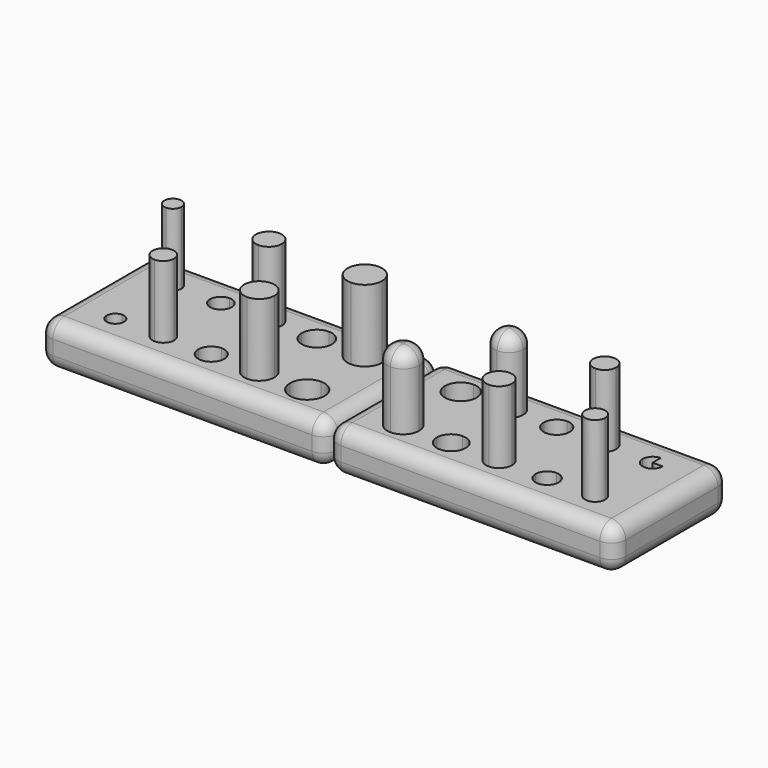
from build123d import *

# Parameters (mm, degrees)
F1_DEPTH = 3
F2_DEPTH = 5
F3_R     = 1
F4_DEPTH = 5
F5_DEPTH = 3
F6_R     = 1
F7_R     = 1


# Not quite as in the source:
# - a feature names something its author has since deleted; it is built from what else it names


with BuildPart() as f1:
    # F0 (on Top) → F1 (new body)
    with BuildSketch(Plane.XY):
        with BuildLine():
            Line((10, 0), (10, 2.5))
            Line((10, 2.5), (6.6666666667, 2.5))
            Line((6.6666666667, 2.5), (6.6666666667, 1.2))
            ThreePointArc((6.6666666667, 1.2), (7.5151948041, 0.8485281374), (7.8666666667, 0))
            Line((7.8666666667, 0), (10, 0))
        make_face()
        with BuildLine():
            Line((-6.6666666667, 0.6), (-6.6666666667, 2.5))
            Line((-6.6666666667, 2.5), (-10, 2.5))
            Line((-10, 2.5), (-10, 0))
            Line((-10, 0), (-7.2666666667, 0))
            ThreePointArc((-7.2666666667, 0), (-7.0909307354, 0.4242640687), (-6.6666666667, 0.6))
        make_face()
        with BuildLine():
            Line((10, -7.5), (10, -5))
            Line((10, -5), (7.8666666667, -5))
            ThreePointArc((7.8666666667, -5), (7.5151948041, -5.8485281374), (6.6666666667, -6.2))
            Line((6.6666666667, -6.2), (6.6666666667, -7.5))
            Line((6.6666666667, -7.5), (10, -7.5))
        make_face()
        with BuildLine():
            Line((-7.2666666667, -5), (-10, -5))
            Line((-10, -5), (-10, -7.5))
            Line((-10, -7.5), (-6.6666666667, -7.5))
            Line((-6.6666666667, -7.5), (-6.6666666667, -5.6))
            ThreePointArc((-6.6666666667, -5.6), (-7.0909307354, -5.4242640687), (-7.2666666667, -5))
        make_face()
        with BuildLine():
            Line((10, -2.5), (10, 0))
            Line((10, 0), (7.8666666667, 0))
            ThreePointArc((7.8666666667, 0), (7.5151948041, -0.8485281374), (6.6666666667, -1.2))
            Line((6.6666666667, -1.2), (6.6666666667, -2.5))
            Line((6.6666666667, -2.5), (10, -2.5))
        make_face()
        with BuildLine():
            Line((10, -5), (10, -2.5))
            Line((10, -2.5), (6.6666666667, -2.5))
            Line((6.6666666667, -2.5), (6.6666666667, -3.8))
            ThreePointArc((6.6666666667, -3.8), (7.5151948041, -4.1514718626), (7.8666666667, -5))
            Line((7.8666666667, -5), (10, -5))
        make_face()
        with BuildLine():
            Line((-7.2666666667, 0), (-10, 0))
            Line((-10, 0), (-10, -2.5))
            Line((-10, -2.5), (-6.6666666667, -2.5))
            Line((-6.6666666667, -2.5), (-6.6666666667, -0.6))
            ThreePointArc((-6.6666666667, -0.6), (-7.0909307354, -0.4242640687), (-7.2666666667, 0))
        make_face()
        with BuildLine():
            Line((-6.6666666667, -4.4), (-6.6666666667, -2.5))
            Line((-6.6666666667, -2.5), (-10, -2.5))
            Line((-10, -2.5), (-10, -5))
            Line((-10, -5), (-7.2666666667, -5))
            ThreePointArc((-7.2666666667, -5), (-7.0909307354, -4.5757359313), (-6.6666666667, -4.4))
        make_face()
        with BuildLine():
            Line((6.6666666667, 1.2), (6.6666666667, 2.5))
            Line((6.6666666667, 2.5), (3.3333333333, 2.5))
            Line((3.3333333333, 2.5), (3.3333333333, 1.05))
            ThreePointArc((3.3333333333, 1.05), (4.0757954536, 0.7424621202), (4.3833333333, 0))
            Line((4.3833333333, 0), (5.4666666667, 0))
            ThreePointArc((5.4666666667, 0), (5.8181385292, 0.8485281374), (6.6666666667, 1.2))
        make_face()
        with BuildLine():
            Line((3.3333333333, 1.05), (3.3333333333, 2.5))
            Line((3.3333333333, 2.5), (0, 2.5))
            Line((0, 2.5), (0, 0.9))
            ThreePointArc((0, 0.9), (0.6363961031, 0.6363961031), (0.9, 0))
            Line((0.9, 0), (2.2833333333, 0))
            ThreePointArc((2.2833333333, 0), (2.5908712131, 0.7424621202), (3.3333333333, 1.05))
        make_face()
        with BuildLine():
            Line((0, 0.9), (0, 2.5))
            Line((0, 2.5), (-3.3333333333, 2.5))
            Line((-3.3333333333, 2.5), (-3.3333333333, 0.75))
            ThreePointArc((-3.3333333333, 0.75), (-2.8030032474, 0.5303300859), (-2.5833333333, 0))
            Line((-2.5833333333, 0), (-0.9, 0))
            ThreePointArc((-0.9, 0), (-0.6363961031, 0.6363961031), (0, 0.9))
        make_face()
        with BuildLine():
            Line((-3.3333333333, 0.75), (-3.3333333333, 2.5))
            Line((-3.3333333333, 2.5), (-6.6666666667, 2.5))
            Line((-6.6666666667, 2.5), (-6.6666666667, 0.6))
            ThreePointArc((-6.6666666667, 0.6), (-6.242402598, 0.4242640687), (-6.0666666667, 0))
            Line((-6.0666666667, 0), (-4.0833333333, 0))
            ThreePointArc((-4.0833333333, 0), (-3.8636634192, 0.5303300859), (-3.3333333333, 0.75))
        make_face()
        with BuildLine():
            ThreePointArc((3.3333333333, -6.05), (2.5908712131, -5.7424621202), (2.2833333333, -5))
            Line((2.2833333333, -5), (0.9, -5))
            ThreePointArc((0.9, -5), (0.6363961031, -5.6363961031), (0, -5.9))
            Line((0, -5.9), (0, -7.5))
            Line((0, -7.5), (3.3333333333, -7.5))
            Line((3.3333333333, -7.5), (3.3333333333, -6.05))
        make_face()
        with BuildLine():
            ThreePointArc((-3.3333333333, -5.75), (-3.8636634192, -5.5303300859), (-4.0833333333, -5))
            Line((-4.0833333333, -5), (-6.0666666667, -5))
            ThreePointArc((-6.0666666667, -5), (-6.242402598, -5.4242640687), (-6.6666666667, -5.6))
            Line((-6.6666666667, -5.6), (-6.6666666667, -7.5))
            Line((-6.6666666667, -7.5), (-3.3333333333, -7.5))
            Line((-3.3333333333, -7.5), (-3.3333333333, -5.75))
        make_face()
        with BuildLine():
            ThreePointArc((6.6666666667, -1.2), (5.8181385292, -0.8485281374), (5.4666666667, 0))
            Line((5.4666666667, 0), (4.3833333333, 0))
            ThreePointArc((4.3833333333, 0), (4.0757954536, -0.7424621202), (3.3333333333, -1.05))
            Line((3.3333333333, -1.05), (3.3333333333, -2.5))
            Line((3.3333333333, -2.5), (6.6666666667, -2.5))
            Line((6.6666666667, -2.5), (6.6666666667, -1.2))
        make_face()
        with BuildLine():
            ThreePointArc((3.3333333333, -1.05), (2.5908712131, -0.7424621202), (2.2833333333, 0))
            Line((2.2833333333, 0), (0.9, 0))
            ThreePointArc((0.9, 0), (0.6363961031, -0.6363961031), (0, -0.9))
            Line((0, -0.9), (0, -2.5))
            Line((0, -2.5), (3.3333333333, -2.5))
            Line((3.3333333333, -2.5), (3.3333333333, -1.05))
        make_face()
        with BuildLine():
            ThreePointArc((0, -0.9), (-0.6363961031, -0.6363961031), (-0.9, 0))
            Line((-0.9, 0), (-2.5833333333, 0))
            ThreePointArc((-2.5833333333, 0), (-2.8030032474, -0.5303300859), (-3.3333333333, -0.75))
            Line((-3.3333333333, -0.75), (-3.3333333333, -2.5))
            Line((-3.3333333333, -2.5), (0, -2.5))
            Line((0, -2.5), (0, -0.9))
        make_face()
        with BuildLine():
            ThreePointArc((-3.3333333333, -0.75), (-3.8636634192, -0.5303300859), (-4.0833333333, 0))
            Line((-4.0833333333, 0), (-6.0666666667, 0))
            ThreePointArc((-6.0666666667, 0), (-6.242402598, -0.4242640687), (-6.6666666667, -0.6))
            Line((-6.6666666667, -0.6), (-6.6666666667, -2.5))
            Line((-6.6666666667, -2.5), (-3.3333333333, -2.5))
            Line((-3.3333333333, -2.5), (-3.3333333333, -0.75))
        make_face()
        with BuildLine():
            Line((0, -4.1), (0, -2.5))
            Line((0, -2.5), (-3.3333333333, -2.5))
            Line((-3.3333333333, -2.5), (-3.3333333333, -4.25))
            ThreePointArc((-3.3333333333, -4.25), (-2.8030032474, -4.4696699141), (-2.5833333333, -5))
            Line((-2.5833333333, -5), (-0.9, -5))
            ThreePointArc((-0.9, -5), (-0.6363961031, -4.3636038969), (0, -4.1))
        make_face()
        with BuildLine():
            Line((3.3333333333, -3.95), (3.3333333333, -2.5))
            Line((3.3333333333, -2.5), (0, -2.5))
            Line((0, -2.5), (0, -4.1))
            ThreePointArc((0, -4.1), (0.6363961031, -4.3636038969), (0.9, -5))
            Line((0.9, -5), (2.2833333333, -5))
            ThreePointArc((2.2833333333, -5), (2.5908712131, -4.2575378798), (3.3333333333, -3.95))
        make_face()
        with BuildLine():
            Line((6.6666666667, -3.8), (6.6666666667, -2.5))
            Line((6.6666666667, -2.5), (3.3333333333, -2.5))
            Line((3.3333333333, -2.5), (3.3333333333, -3.95))
            ThreePointArc((3.3333333333, -3.95), (4.0757954536, -4.2575378798), (4.3833333333, -5))
            Line((4.3833333333, -5), (5.4666666667, -5))
            ThreePointArc((5.4666666667, -5), (5.8181385292, -4.1514718626), (6.6666666667, -3.8))
        make_face()
        with BuildLine():
            ThreePointArc((6.6666666667, -6.2), (5.8181385292, -5.8485281374), (5.4666666667, -5))
            Line((5.4666666667, -5), (4.3833333333, -5))
            ThreePointArc((4.3833333333, -5), (4.0757954536, -5.7424621202), (3.3333333333, -6.05))
            Line((3.3333333333, -6.05), (3.3333333333, -7.5))
            Line((3.3333333333, -7.5), (6.6666666667, -7.5))
            Line((6.6666666667, -7.5), (6.6666666667, -6.2))
        make_face()
        with BuildLine():
            ThreePointArc((0, -5.9), (-0.6363961031, -5.6363961031), (-0.9, -5))
            Line((-0.9, -5), (-2.5833333333, -5))
            ThreePointArc((-2.5833333333, -5), (-2.8030032474, -5.5303300859), (-3.3333333333, -5.75))
            Line((-3.3333333333, -5.75), (-3.3333333333, -7.5))
            Line((-3.3333333333, -7.5), (0, -7.5))
            Line((0, -7.5), (0, -5.9))
        make_face()
        with BuildLine():
            Line((-6.6666666667, -0.6), (-6.6666666667, 0))
            Line((-6.6666666667, 0), (-7.2666666667, 0))
            ThreePointArc((-7.2666666667, 0), (-7.0909307354, -0.4242640687), (-6.6666666667, -0.6))
        make_face()
        with BuildLine():
            Line((-6.0666666667, 0), (-6.6666666667, 0))
            Line((-6.6666666667, 0), (-6.6666666667, -0.6))
            ThreePointArc((-6.6666666667, -0.6), (-6.242402598, -0.4242640687), (-6.0666666667, 0))
        make_face()
        with BuildLine():
            ThreePointArc((-6.0666666667, 0), (-6.242402598, 0.4242640687), (-6.6666666667, 0.6))
            Line((-6.6666666667, 0.6), (-6.6666666667, 0))
            Line((-6.6666666667, 0), (-6.0666666667, 0))
        make_face()
        with BuildLine():
            Line((-6.6666666667, 0), (-6.6666666667, 0.6))
            ThreePointArc((-6.6666666667, 0.6), (-7.0909307354, 0.4242640687), (-7.2666666667, 0))
            Line((-7.2666666667, 0), (-6.6666666667, 0))
        make_face()
        with BuildLine():
            Line((0, 0), (0, 0.9))
            ThreePointArc((0, 0.9), (-0.6363961031, 0.6363961031), (-0.9, 0))
            Line((-0.9, 0), (0, 0))
        make_face()
        with BuildLine():
            ThreePointArc((0, -0.9), (0.6363961031, -0.6363961031), (0.9, 0))
            Line((0.9, 0), (0, 0))
            Line((0, 0), (0, -0.9))
        make_face()
        with BuildLine():
            ThreePointArc((0.9, 0), (0.6363961031, 0.6363961031), (0, 0.9))
            Line((0, 0.9), (0, 0))
            Line((0, 0), (0.9, 0))
        make_face()
        with BuildLine():
            ThreePointArc((7.8666666667, 0), (7.5151948041, 0.8485281374), (6.6666666667, 1.2))
            Line((6.6666666667, 1.2), (6.6666666667, 0))
            Line((6.6666666667, 0), (7.8666666667, 0))
        make_face()
        with BuildLine():
            ThreePointArc((6.6666666667, -1.2), (7.5151948041, -0.8485281374), (7.8666666667, 0))
            Line((7.8666666667, 0), (6.6666666667, 0))
            Line((6.6666666667, 0), (6.6666666667, -1.2))
        make_face()
        with BuildLine():
            Line((6.6666666667, -1.2), (6.6666666667, 0))
            Line((6.6666666667, 0), (5.4666666667, 0))
            ThreePointArc((5.4666666667, 0), (5.8181385292, -0.8485281374), (6.6666666667, -1.2))
        make_face()
        with BuildLine():
            Line((6.6666666667, 0), (6.6666666667, 1.2))
            ThreePointArc((6.6666666667, 1.2), (5.8181385292, 0.8485281374), (5.4666666667, 0))
            Line((5.4666666667, 0), (6.6666666667, 0))
        make_face()
        with BuildLine():
            Line((0, 0), (-0.9, 0))
            ThreePointArc((-0.9, 0), (-0.6363961031, -0.6363961031), (0, -0.9))
            Line((0, -0.9), (0, 0))
        make_face()
        with BuildLine():
            Line((3.3333333333, -6.05), (3.3333333333, -5))
            Line((3.3333333333, -5), (2.2833333333, -5))
            ThreePointArc((2.2833333333, -5), (2.5908712131, -5.7424621202), (3.3333333333, -6.05))
        make_face()
        with BuildLine():
            Line((3.3333333333, -5), (3.3333333333, -3.95))
            ThreePointArc((3.3333333333, -3.95), (2.5908712131, -4.2575378798), (2.2833333333, -5))
            Line((2.2833333333, -5), (3.3333333333, -5))
        make_face()
        with BuildLine():
            ThreePointArc((4.3833333333, -5), (4.0757954536, -4.2575378798), (3.3333333333, -3.95))
            Line((3.3333333333, -3.95), (3.3333333333, -5))
            Line((3.3333333333, -5), (4.3833333333, -5))
        make_face()
        with BuildLine():
            Line((4.3833333333, -5), (3.3333333333, -5))
            Line((3.3333333333, -5), (3.3333333333, -6.05))
            ThreePointArc((3.3333333333, -6.05), (4.0757954536, -5.7424621202), (4.3833333333, -5))
        make_face()
        with BuildLine():
            Line((-2.5833333333, -5), (-3.3333333333, -5))
            Line((-3.3333333333, -5), (-3.3333333333, -5.75))
            ThreePointArc((-3.3333333333, -5.75), (-2.8030032474, -5.5303300859), (-2.5833333333, -5))
        make_face()
        with BuildLine():
            Line((-3.3333333333, -5.75), (-3.3333333333, -5))
            Line((-3.3333333333, -5), (-4.0833333333, -5))
            ThreePointArc((-4.0833333333, -5), (-3.8636634192, -5.5303300859), (-3.3333333333, -5.75))
        make_face()
        with BuildLine():
            ThreePointArc((-2.5833333333, -5), (-2.8030032474, -4.4696699141), (-3.3333333333, -4.25))
            Line((-3.3333333333, -4.25), (-3.3333333333, -5))
            Line((-3.3333333333, -5), (-2.5833333333, -5))
        make_face()
        with BuildLine():
            Line((-3.3333333333, -4.25), (-3.3333333333, -2.5))
            Line((-3.3333333333, -2.5), (-6.6666666667, -2.5))
            Line((-6.6666666667, -2.5), (-6.6666666667, -4.4))
            ThreePointArc((-6.6666666667, -4.4), (-6.242402598, -4.5757359313), (-6.0666666667, -5))
            Line((-6.0666666667, -5), (-4.0833333333, -5))
            ThreePointArc((-4.0833333333, -5), (-3.8636634192, -4.4696699141), (-3.3333333333, -4.25))
        make_face()
        with BuildLine():
            Line((-3.3333333333, -5), (-3.3333333333, -4.25))
            ThreePointArc((-3.3333333333, -4.25), (-3.8636634192, -4.4696699141), (-4.0833333333, -5))
            Line((-4.0833333333, -5), (-3.3333333333, -5))
        make_face()
    extrude(amount=-F1_DEPTH)

    # F0 (on Top) → F2 (join)
    with BuildSketch(Plane.XY):
        with BuildLine():
            Line((0, 0), (-0.9, 0))
            ThreePointArc((-0.9, 0), (-0.6363961031, -0.6363961031), (0, -0.9))
            Line((0, -0.9), (0, 0))
        make_face()
        with BuildLine():
            Line((0, 0), (0, 0.9))
            ThreePointArc((0, 0.9), (-0.6363961031, 0.6363961031), (-0.9, 0))
            Line((-0.9, 0), (0, 0))
        make_face()
        with BuildLine():
            ThreePointArc((0, -0.9), (0.6363961031, -0.6363961031), (0.9, 0))
            Line((0.9, 0), (0, 0))
            Line((0, 0), (0, -0.9))
        make_face()
        with BuildLine():
            ThreePointArc((0.9, 0), (0.6363961031, 0.6363961031), (0, 0.9))
            Line((0, 0.9), (0, 0))
            Line((0, 0), (0.9, 0))
        make_face()
        with BuildLine():
            ThreePointArc((-2.5833333333, -5), (-2.8030032474, -4.4696699141), (-3.3333333333, -4.25))
            Line((-3.3333333333, -4.25), (-3.3333333333, -5))
            Line((-3.3333333333, -5), (-2.5833333333, -5))
        make_face()
        with BuildLine():
            Line((-2.5833333333, -5), (-3.3333333333, -5))
            Line((-3.3333333333, -5), (-3.3333333333, -5.75))
            ThreePointArc((-3.3333333333, -5.75), (-2.8030032474, -5.5303300859), (-2.5833333333, -5))
        make_face()
        with BuildLine():
            Line((-3.3333333333, -5.75), (-3.3333333333, -5))
            Line((-3.3333333333, -5), (-4.0833333333, -5))
            ThreePointArc((-4.0833333333, -5), (-3.8636634192, -5.5303300859), (-3.3333333333, -5.75))
        make_face()
        with BuildLine():
            Line((-3.3333333333, -5), (-3.3333333333, -4.25))
            ThreePointArc((-3.3333333333, -4.25), (-3.8636634192, -4.4696699141), (-4.0833333333, -5))
            Line((-4.0833333333, -5), (-3.3333333333, -5))
        make_face()
        with BuildLine():
            ThreePointArc((-6.0666666667, 0), (-6.242402598, 0.4242640687), (-6.6666666667, 0.6))
            Line((-6.6666666667, 0.6), (-6.6666666667, 0))
            Line((-6.6666666667, 0), (-6.0666666667, 0))
        make_face()
        with BuildLine():
            Line((-6.6666666667, 0), (-6.6666666667, 0.6))
            ThreePointArc((-6.6666666667, 0.6), (-7.0909307354, 0.4242640687), (-7.2666666667, 0))
            Line((-7.2666666667, 0), (-6.6666666667, 0))
        make_face()
        with BuildLine():
            Line((-6.6666666667, -0.6), (-6.6666666667, 0))
            Line((-6.6666666667, 0), (-7.2666666667, 0))
            ThreePointArc((-7.2666666667, 0), (-7.0909307354, -0.4242640687), (-6.6666666667, -0.6))
        make_face()
        with BuildLine():
            Line((-6.0666666667, 0), (-6.6666666667, 0))
            Line((-6.6666666667, 0), (-6.6666666667, -0.6))
            ThreePointArc((-6.6666666667, -0.6), (-6.242402598, -0.4242640687), (-6.0666666667, 0))
        make_face()
        with BuildLine():
            Line((3.3333333333, -5), (3.3333333333, -3.95))
            ThreePointArc((3.3333333333, -3.95), (2.5908712131, -4.2575378798), (2.2833333333, -5))
            Line((2.2833333333, -5), (3.3333333333, -5))
        make_face()
        with BuildLine():
            Line((3.3333333333, -6.05), (3.3333333333, -5))
            Line((3.3333333333, -5), (2.2833333333, -5))
            ThreePointArc((2.2833333333, -5), (2.5908712131, -5.7424621202), (3.3333333333, -6.05))
        make_face()
        with BuildLine():
            Line((4.3833333333, -5), (3.3333333333, -5))
            Line((3.3333333333, -5), (3.3333333333, -6.05))
            ThreePointArc((3.3333333333, -6.05), (4.0757954536, -5.7424621202), (4.3833333333, -5))
        make_face()
        with BuildLine():
            ThreePointArc((4.3833333333, -5), (4.0757954536, -4.2575378798), (3.3333333333, -3.95))
            Line((3.3333333333, -3.95), (3.3333333333, -5))
            Line((3.3333333333, -5), (4.3833333333, -5))
        make_face()
        with BuildLine():
            Line((6.6666666667, -1.2), (6.6666666667, 0))
            Line((6.6666666667, 0), (5.4666666667, 0))
            ThreePointArc((5.4666666667, 0), (5.8181385292, -0.8485281374), (6.6666666667, -1.2))
        make_face()
        with BuildLine():
            Line((6.6666666667, 0), (6.6666666667, 1.2))
            ThreePointArc((6.6666666667, 1.2), (5.8181385292, 0.8485281374), (5.4666666667, 0))
            Line((5.4666666667, 0), (6.6666666667, 0))
        make_face()
        with BuildLine():
            ThreePointArc((7.8666666667, 0), (7.5151948041, 0.8485281374), (6.6666666667, 1.2))
            Line((6.6666666667, 1.2), (6.6666666667, 0))
            Line((6.6666666667, 0), (7.8666666667, 0))
        make_face()
        with BuildLine():
            ThreePointArc((6.6666666667, -1.2), (7.5151948041, -0.8485281374), (7.8666666667, 0))
            Line((7.8666666667, 0), (6.6666666667, 0))
            Line((6.6666666667, 0), (6.6666666667, -1.2))
        make_face()
    extrude(amount=F2_DEPTH)

    # F3
    f3_edges = [f1.edges().sort_by_distance(p)[0] for p in [
        (-10, 2.5, -1.5),
        (-10, -7.5, -1.5),
        (-10, -2.5, 0),
        (-10, -2.5, -3),
        (10, -7.5, -1.5),
        (0, -7.5, 0),
        (0, -7.5, -3),
        (10, 2.5, -1.5),
        (0, 2.5, 0),
        (0, 2.5, -3),
        (10, -2.5, 0),
        (10, -2.5, -3),
    ]]
    fillet(f3_edges, radius=F3_R)


with BuildPart() as f4:
    # F0 (on Top) → F4 (new body)
    with BuildSketch(Plane.XY):
        with BuildLine():
            ThreePointArc((24.1333333333, 0), (23.8990187583, 0.5656854249), (23.3333333333, 0.8))
            ThreePointArc((23.3333333333, 0.8), (22.7676479084, 0.5656854249), (22.5333333333, 0))
            ThreePointArc((22.5333333333, 0), (22.7676479084, -0.5656854249), (23.3333333333, -0.8))
            ThreePointArc((23.3333333333, -0.8), (23.8990187583, -0.5656854249), (24.1333333333, 0))
        make_face()
    extrude(amount=F4_DEPTH)



with BuildPart() as f4b:
    # F0 (on Top) → F4, piece 2 (new body)
    with BuildSketch(Plane.XY):
        with BuildLine():
            ThreePointArc((20.9, -5), (20.6363961031, -4.3636038969), (20, -4.1))
            ThreePointArc((20, -4.1), (19.3636038969, -4.3636038969), (19.1, -5))
            ThreePointArc((19.1, -5), (19.3636038969, -5.6363961031), (20, -5.9))
            ThreePointArc((20, -5.9), (20.6363961031, -5.6363961031), (20.9, -5))
        make_face()
    extrude(amount=F4_DEPTH)


with BuildPart() as f4c:
    # F0 (on Top) → F4, piece 3 (new body)
    with BuildSketch(Plane.XY):
        with BuildLine():
            ThreePointArc((17.6666666667, 0), (17.3737734479, 0.7071067812), (16.6666666667, 1))
            ThreePointArc((16.6666666667, 1), (15.6666666667, 0), (16.6666666667, -1))
            ThreePointArc((16.6666666667, -1), (17.3737734479, -0.7071067812), (17.6666666667, 0))
        make_face()
    extrude(amount=F4_DEPTH)


with BuildPart() as f4d:
    # F0 (on Top) → F4, piece 4 (new body)
    with BuildSketch(Plane.XY):
        with BuildLine():
            ThreePointArc((13.3333333333, -3.9), (12.555515874, -4.2221825407), (12.2333333333, -5))
            ThreePointArc((12.2333333333, -5), (12.555515874, -5.7778174593), (13.3333333333, -6.1))
            ThreePointArc((13.3333333333, -6.1), (14.1111507926, -5.7778174593), (14.4333333333, -5))
            ThreePointArc((14.4333333333, -5), (14.1111507926, -4.2221825407), (13.3333333333, -3.9))
        make_face()
    extrude(amount=F4_DEPTH)


with BuildPart() as f4e:
    # F0 (on Top) → F4, piece 5 (new body)
    with BuildSketch(Plane.XY):
        with BuildLine():
            ThreePointArc((27.3666666667, -5), (27.1616414135, -4.5050252532), (26.6666666667, -4.3))
            ThreePointArc((26.6666666667, -4.3), (26.1716919198, -4.5050252532), (25.9666666667, -5))
            ThreePointArc((25.9666666667, -5), (26.6666666667, -5.7), (27.3666666667, -5))
        make_face()
    extrude(amount=F4_DEPTH)


with BuildPart() as f4_1:
    add(f4.part)

    add(f4b.part)  # F5 merges F4b

    add(f4c.part)  # F5 merges F4c

    add(f4d.part)  # F5 merges F4d

    add(f4e.part)  # F5 merges F4e
    # F0 (on Top) → F5 (join)
    with BuildSketch(Plane.XY):
        with BuildLine():
            Line((23.3333333333, 2.5), (20, 2.5))
            Line((20, 2.5), (20, 0.9))
            ThreePointArc((20, 0.9), (20.6363961031, 0.6363961031), (20.9, 0))
            Line((20.9, 0), (22.5333333333, 0))
            ThreePointArc((22.5333333333, 0), (22.7676479084, 0.5656854249), (23.3333333333, 0.8))
            Line((23.3333333333, 0.8), (23.3333333333, 2.5))
        make_face()
        with BuildLine():
            Line((12.2333333333, -5), (10, -5))
            Line((10, -5), (10, -7.5))
            Line((10, -7.5), (13.3333333333, -7.5))
            Line((13.3333333333, -7.5), (13.3333333333, -6.1))
            ThreePointArc((13.3333333333, -6.1), (12.555515874, -5.7778174593), (12.2333333333, -5))
        make_face()
        with BuildLine():
            Line((16.6666666667, -2.5), (13.3333333333, -2.5))
            Line((13.3333333333, -2.5), (13.3333333333, -3.9))
            ThreePointArc((13.3333333333, -3.9), (14.1111507926, -4.2221825407), (14.4333333333, -5))
            Line((14.4333333333, -5), (15.6666666667, -5))
            ThreePointArc((15.6666666667, -5), (15.9595598855, -4.2928932188), (16.6666666667, -4))
            Line((16.6666666667, -4), (16.6666666667, -2.5))
        make_face()
        with BuildLine():
            Line((20, -5.9), (20, -7.5))
            Line((20, -7.5), (30, -7.5))
            Line((30, -7.5), (30, -5))
            Line((30, -5), (27.3666666667, -5))
            ThreePointArc((27.3666666667, -5), (26.6666666667, -5.7), (25.9666666667, -5))
            Line((25.9666666667, -5), (24.1333333333, -5))
            ThreePointArc((24.1333333333, -5), (23.3333333333, -5.8), (22.5333333333, -5))
            Line((22.5333333333, -5), (20.9, -5))
            ThreePointArc((20.9, -5), (20.6363961031, -5.6363961031), (20, -5.9))
        make_face()
        with BuildLine():
            Line((12.2333333333, 0), (10, 0))
            Line((10, 0), (10, -2.5))
            Line((10, -2.5), (13.3333333333, -2.5))
            Line((13.3333333333, -2.5), (13.3333333333, -1.1))
            ThreePointArc((13.3333333333, -1.1), (12.555515874, -0.7778174593), (12.2333333333, 0))
        make_face()
        with BuildLine():
            ThreePointArc((27.3666666667, 0), (27.1616414135, 0.4949747468), (26.6666666667, 0.7))
            Line((26.6666666667, 0.7), (26.6666666667, 0))
            Line((26.6666666667, 0), (27.3666666667, 0))
        make_face()
        with BuildLine():
            ThreePointArc((20.9, -5), (20.6363961031, -4.3636038969), (20, -4.1))
            ThreePointArc((20, -4.1), (19.3636038969, -4.3636038969), (19.1, -5))
            ThreePointArc((19.1, -5), (19.3636038969, -5.6363961031), (20, -5.9))
            ThreePointArc((20, -5.9), (20.6363961031, -5.6363961031), (20.9, -5))
        make_face()
        with BuildLine():
            Line((13.3333333333, -2.5), (10, -2.5))
            Line((10, -2.5), (10, -5))
            Line((10, -5), (12.2333333333, -5))
            ThreePointArc((12.2333333333, -5), (12.555515874, -4.2221825407), (13.3333333333, -3.9))
            Line((13.3333333333, -3.9), (13.3333333333, -2.5))
        make_face()
        with BuildLine():
            Line((30, -2.5), (26.6666666667, -2.5))
            Line((26.6666666667, -2.5), (26.6666666667, -4.3))
            ThreePointArc((26.6666666667, -4.3), (27.1616414135, -4.5050252532), (27.3666666667, -5))
            Line((27.3666666667, -5), (30, -5))
            Line((30, -5), (30, -2.5))
        make_face()
        with BuildLine():
            Line((23.3333333333, -0.8), (23.3333333333, -2.5))
            Line((23.3333333333, -2.5), (26.6666666667, -2.5))
            Line((26.6666666667, -2.5), (30, -2.5))
            Line((30, -2.5), (30, 0))
            Line((30, 0), (27.3666666667, 0))
            ThreePointArc((27.3666666667, 0), (26.6666666667, -0.7), (25.9666666667, 0))
            Line((25.9666666667, 0), (24.1333333333, 0))
            ThreePointArc((24.1333333333, 0), (23.8990187583, -0.5656854249), (23.3333333333, -0.8))
        make_face()
        with BuildLine():
            Line((16.6666666667, -6), (16.6666666667, -7.5))
            Line((16.6666666667, -7.5), (20, -7.5))
            Line((20, -7.5), (20, -5.9))
            ThreePointArc((20, -5.9), (19.3636038969, -5.6363961031), (19.1, -5))
            Line((19.1, -5), (17.6666666667, -5))
            ThreePointArc((17.6666666667, -5), (17.3737734479, -5.7071067812), (16.6666666667, -6))
        make_face()
        with BuildLine():
            ThreePointArc((24.1333333333, 0), (23.8990187583, 0.5656854249), (23.3333333333, 0.8))
            ThreePointArc((23.3333333333, 0.8), (22.7676479084, 0.5656854249), (22.5333333333, 0))
            ThreePointArc((22.5333333333, 0), (22.7676479084, -0.5656854249), (23.3333333333, -0.8))
            ThreePointArc((23.3333333333, -0.8), (23.8990187583, -0.5656854249), (24.1333333333, 0))
        make_face()
        with BuildLine():
            ThreePointArc((17.6666666667, 0), (17.3737734479, 0.7071067812), (16.6666666667, 1))
            ThreePointArc((16.6666666667, 1), (15.6666666667, 0), (16.6666666667, -1))
            ThreePointArc((16.6666666667, -1), (17.3737734479, -0.7071067812), (17.6666666667, 0))
        make_face()
        with BuildLine():
            Line((13.3333333333, -6.1), (13.3333333333, -7.5))
            Line((13.3333333333, -7.5), (16.6666666667, -7.5))
            Line((16.6666666667, -7.5), (16.6666666667, -6))
            ThreePointArc((16.6666666667, -6), (15.9595598855, -5.7071067812), (15.6666666667, -5))
            Line((15.6666666667, -5), (14.4333333333, -5))
            ThreePointArc((14.4333333333, -5), (14.1111507926, -5.7778174593), (13.3333333333, -6.1))
        make_face()
        with BuildLine():
            Line((26.6666666667, -2.5), (23.3333333333, -2.5))
            Line((23.3333333333, -2.5), (23.3333333333, -4.2))
            ThreePointArc((23.3333333333, -4.2), (23.8990187583, -4.4343145751), (24.1333333333, -5))
            Line((24.1333333333, -5), (25.9666666667, -5))
            ThreePointArc((25.9666666667, -5), (26.1716919198, -4.5050252532), (26.6666666667, -4.3))
            Line((26.6666666667, -4.3), (26.6666666667, -2.5))
        make_face()
        with BuildLine():
            Line((16.6666666667, -1), (16.6666666667, -2.5))
            Line((16.6666666667, -2.5), (20, -2.5))
            Line((20, -2.5), (20, -0.9))
            ThreePointArc((20, -0.9), (19.3636038969, -0.6363961031), (19.1, 0))
            Line((19.1, 0), (17.6666666667, 0))
            ThreePointArc((17.6666666667, 0), (17.3737734479, -0.7071067812), (16.6666666667, -1))
        make_face()
        with BuildLine():
            Line((23.3333333333, -2.5), (20, -2.5))
            Line((20, -2.5), (20, -4.1))
            ThreePointArc((20, -4.1), (20.6363961031, -4.3636038969), (20.9, -5))
            Line((20.9, -5), (22.5333333333, -5))
            ThreePointArc((22.5333333333, -5), (22.7676479084, -4.4343145751), (23.3333333333, -4.2))
            Line((23.3333333333, -4.2), (23.3333333333, -2.5))
        make_face()
        with BuildLine():
            Line((26.6666666667, 2.5), (23.3333333333, 2.5))
            Line((23.3333333333, 2.5), (23.3333333333, 0.8))
            ThreePointArc((23.3333333333, 0.8), (23.8990187583, 0.5656854249), (24.1333333333, 0))
            Line((24.1333333333, 0), (25.9666666667, 0))
            ThreePointArc((25.9666666667, 0), (26.1716919198, 0.4949747468), (26.6666666667, 0.7))
            Line((26.6666666667, 0.7), (26.6666666667, 2.5))
        make_face()
        with BuildLine():
            Line((30, 2.5), (26.6666666667, 2.5))
            Line((26.6666666667, 2.5), (26.6666666667, 0.7))
            ThreePointArc((26.6666666667, 0.7), (27.1616414135, 0.4949747468), (27.3666666667, 0))
            Line((27.3666666667, 0), (30, 0))
            Line((30, 0), (30, 2.5))
        make_face()
        with BuildLine():
            Line((16.6666666667, 2.5), (13.3333333333, 2.5))
            Line((13.3333333333, 2.5), (13.3333333333, 1.1))
            ThreePointArc((13.3333333333, 1.1), (14.1111507926, 0.7778174593), (14.4333333333, 0))
            ThreePointArc((14.4333333333, 0), (14.1111507926, -0.7778174593), (13.3333333333, -1.1))
            Line((13.3333333333, -1.1), (13.3333333333, -2.5))
            Line((13.3333333333, -2.5), (16.6666666667, -2.5))
            Line((16.6666666667, -2.5), (16.6666666667, -1))
            ThreePointArc((16.6666666667, -1), (15.6666666667, 0), (16.6666666667, 1))
            Line((16.6666666667, 1), (16.6666666667, 2.5))
        make_face()
        with BuildLine():
            Line((20, -2.5), (16.6666666667, -2.5))
            Line((16.6666666667, -2.5), (16.6666666667, -4))
            ThreePointArc((16.6666666667, -4), (17.3737734479, -4.2928932188), (17.6666666667, -5))
            Line((17.6666666667, -5), (19.1, -5))
            ThreePointArc((19.1, -5), (19.3636038969, -4.3636038969), (20, -4.1))
            Line((20, -4.1), (20, -2.5))
        make_face()
        with BuildLine():
            ThreePointArc((27.3666666667, -5), (27.1616414135, -4.5050252532), (26.6666666667, -4.3))
            ThreePointArc((26.6666666667, -4.3), (26.1716919198, -4.5050252532), (25.9666666667, -5))
            ThreePointArc((25.9666666667, -5), (26.6666666667, -5.7), (27.3666666667, -5))
        make_face()
        with BuildLine():
            Line((13.3333333333, 2.5), (10, 2.5))
            Line((10, 2.5), (10, 0))
            Line((10, 0), (12.2333333333, 0))
            ThreePointArc((12.2333333333, 0), (12.555515874, 0.7778174593), (13.3333333333, 1.1))
            Line((13.3333333333, 1.1), (13.3333333333, 2.5))
        make_face()
        with BuildLine():
            Line((20, -0.9), (20, -2.5))
            Line((20, -2.5), (23.3333333333, -2.5))
            Line((23.3333333333, -2.5), (23.3333333333, -0.8))
            ThreePointArc((23.3333333333, -0.8), (22.7676479084, -0.5656854249), (22.5333333333, 0))
            Line((22.5333333333, 0), (20.9, 0))
            ThreePointArc((20.9, 0), (20.6363961031, -0.6363961031), (20, -0.9))
        make_face()
        with BuildLine():
            Line((20, 2.5), (16.6666666667, 2.5))
            Line((16.6666666667, 2.5), (16.6666666667, 1))
            ThreePointArc((16.6666666667, 1), (17.3737734479, 0.7071067812), (17.6666666667, 0))
            Line((17.6666666667, 0), (19.1, 0))
            ThreePointArc((19.1, 0), (19.3636038969, 0.6363961031), (20, 0.9))
            Line((20, 0.9), (20, 2.5))
        make_face()
        with BuildLine():
            ThreePointArc((13.3333333333, -3.9), (12.555515874, -4.2221825407), (12.2333333333, -5))
            ThreePointArc((12.2333333333, -5), (12.555515874, -5.7778174593), (13.3333333333, -6.1))
            ThreePointArc((13.3333333333, -6.1), (14.1111507926, -5.7778174593), (14.4333333333, -5))
            ThreePointArc((14.4333333333, -5), (14.1111507926, -4.2221825407), (13.3333333333, -3.9))
        make_face()
    extrude(amount=-F5_DEPTH)

    # F6
    f6_edges = [f4_1.edges().sort_by_distance(p)[0] for p in [
        (10, 2.5, -1.5),
        (10, -7.5, -1.5),
        (10, -2.5, 0),
        (10, -2.5, -3),
        (30, 2.5, -1.5),
        (20, 2.5, 0),
        (20, 2.5, -3),
        (30, -7.5, -1.5),
        (30, -2.5, 0),
        (30, -2.5, -3),
        (20, -7.5, 0),
        (20, -7.5, -3),
    ]]
    fillet(f6_edges, radius=F6_R)

    # F7
    f7_edges = [f4_1.edges().sort_by_distance(p)[0] for p in [
        (13.333333, -3.9, 5),
        (16.666667, 1, 5),
    ]]
    fillet(f7_edges, radius=F7_R)


solid = Compound([f1.part, f4_1.part])
